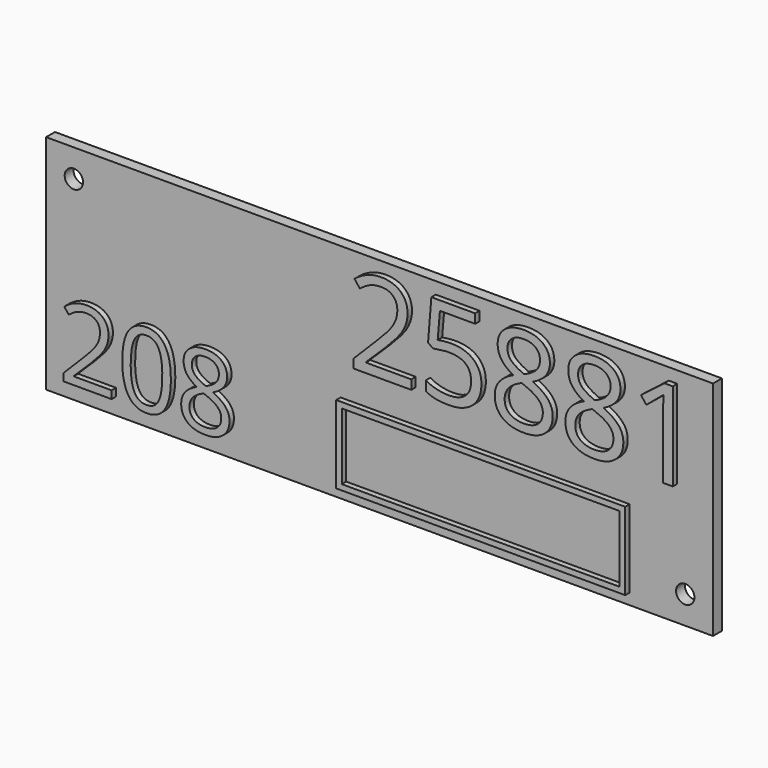
from build123d import *

# Parameters (mm, degrees)
F0_W         = 120
F0_H         = 40
F1_DEPTH     = 2
F3_D         = 3.3
F4_TEXT_SIZE = 22.2157940411
F5_DEPTH     = 1
F6_TEXT_SIZE = 18.5155049272
F7_DEPTH     = 1
F8_W         = 52
F8_H         = 14
F8_W_2       = 49.99999962
F8_H_2       = 11.99999962
F9_DEPTH     = 1


# Not quite as in the source:
# - Text() gives the source's letters only with a copy of the font that has no kerning and outlines rounded to 1/6400 em; it was checked with that copy


with BuildPart() as f1:
    # F0 (on Front) → F1 (new body)
    with BuildSketch(Plane.XZ):
        Rectangle(F0_W, F0_H)
    extrude(amount=F1_DEPTH)

    # F3 (through all)
    with Locations(Plane.XZ.offset(2)):
        with Locations((-55, 15), (55, -15)):
            Hole(F3_D / 2)

    # F4 (on face) → F5 (join)
    with BuildSketch(Plane.XZ.offset(2)):
        with Locations((-5, 2)):
            Text('25881', F4_TEXT_SIZE, font='Open Sans', text_align=(TextAlign.LEFT, TextAlign.BOTTOM))
    extrude(amount=F5_DEPTH)

    # F6 (on face) → F7 (join)
    with BuildSketch(Plane.XZ.offset(2)):
        with Locations((-57, -17)):
            Text('208', F6_TEXT_SIZE, font='Open Sans', text_align=(TextAlign.LEFT, TextAlign.BOTTOM))
    extrude(amount=F7_DEPTH)

    # F8 (on face) → F9 (join)
    with BuildSketch(Plane.XZ.offset(2)):
        with Locations((19, -11)):
            Rectangle(F8_W, F8_H)
        with Locations((19, -11)):
            Rectangle(F8_W_2, F8_H_2, mode=Mode.SUBTRACT)
    extrude(amount=F9_DEPTH)


solid = f1.part
